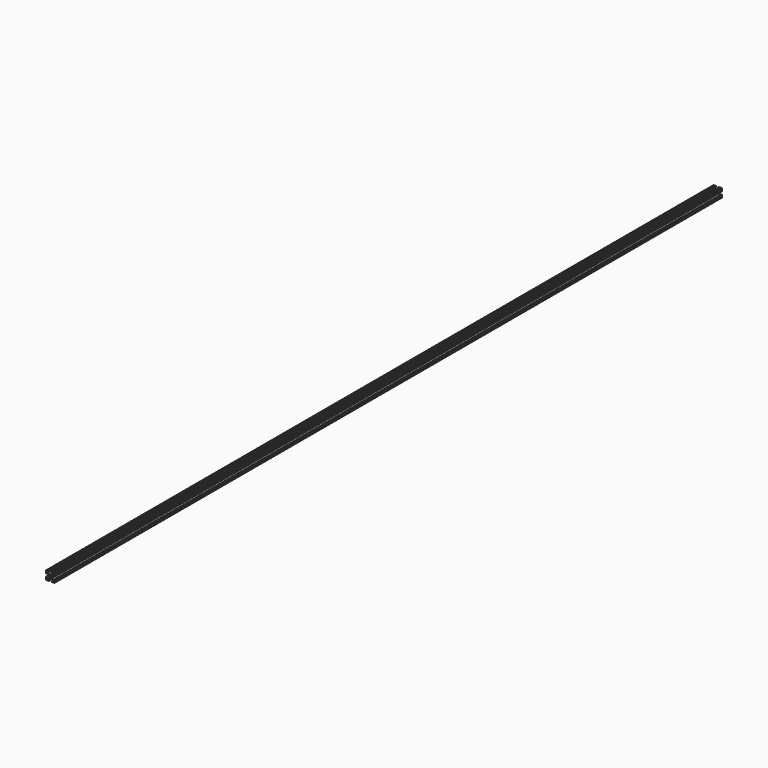
from build123d import *

# Parameters (mm, degrees)
F1_DEPTH    = 2438.4
F2_T1_DEPTH = 2438.4
F2_T3_DEPTH = 2446.3375
F2_T5_DEPTH = 2442.36875


# Not quite as in the source:
# - a fillet or chamfer that OpenCascade refuses, or shapes differently, is made with other operations: its cross-section is extruded or revolved along the edge and cut away or added


with BuildPart() as f1:
    # F0 (on Front) → F1 (new body)
    with BuildSketch(Plane.XZ):
        with BuildLine():
            ThreePointArc((-0.8361427067, 2.2296225996), (0, 2.38125), (0.8361427067, 2.2296225996))
            Line((0.8361427067, 2.2296225996), (3.1853789104, 4.5640625))
            Line((3.1853789104, 4.5640625), (-3.1853789104, 4.5640625))
            Line((-3.1853789104, 4.5640625), (-0.8361427067, 2.2296225996))
        make_face()
        with BuildLine():
            ThreePointArc((-2.2347427098, 0.8223603732), (-1.6889881746, 1.6785918231), (-0.8361427067, 2.2296225996))
            Line((-0.8361427067, 2.2296225996), (-3.1853789104, 4.5640625))
            Line((-3.1853789104, 4.5640625), (-4.5640625, 4.5640625))
            Line((-4.5640625, 4.5640625), (-4.5640625, 3.1376763557))
            Line((-4.5640625, 3.1376763557), (-2.2347427098, 0.8223603732))
        make_face()
        with BuildLine():
            ThreePointArc((-2.2347427098, -0.8223603732), (-2.38125, 0), (-2.2347427098, 0.8223603732))
            Line((-2.2347427098, 0.8223603732), (-4.5640625, 3.1376763557))
            Line((-4.5640625, 3.1376763557), (-4.5640625, -3.1376763557))
            Line((-4.5640625, -3.1376763557), (-2.2347427098, -0.8223603732))
        make_face()
        with BuildLine():
            Line((-3.1853789104, -4.5640625), (-0.8361427067, -2.2296225996))
            ThreePointArc((-0.8361427067, -2.2296225996), (-1.6889881746, -1.6785918231), (-2.2347427098, -0.8223603732))
            Line((-2.2347427098, -0.8223603732), (-4.5640625, -3.1376763557))
            Line((-4.5640625, -3.1376763557), (-4.5640625, -4.5640625))
            Line((-4.5640625, -4.5640625), (-3.1853789104, -4.5640625))
        make_face()
        with BuildLine():
            Line((3.1853789104, -4.5640625), (0.8361427067, -2.2296225996))
            ThreePointArc((0.8361427067, -2.2296225996), (0, -2.38125), (-0.8361427067, -2.2296225996))
            Line((-0.8361427067, -2.2296225996), (-3.1853789104, -4.5640625))
            Line((-3.1853789104, -4.5640625), (3.1853789104, -4.5640625))
        make_face()
        with BuildLine():
            Line((4.5640625, -3.1376763557), (2.2347427098, -0.8223603732))
            ThreePointArc((2.2347427098, -0.8223603732), (1.6889881746, -1.6785918231), (0.8361427067, -2.2296225996))
            Line((0.8361427067, -2.2296225996), (3.1853789104, -4.5640625))
            Line((3.1853789104, -4.5640625), (4.5640625, -4.5640625))
            Line((4.5640625, -4.5640625), (4.5640625, -3.1376763557))
        make_face()
        with BuildLine():
            ThreePointArc((2.2347427098, 0.8223603732), (2.3443370748, 0.4176544533), (2.38125, 0))
            ThreePointArc((2.38125, 0), (2.3443370748, -0.4176544533), (2.2347427098, -0.8223603732))
            Line((2.2347427098, -0.8223603732), (4.5640625, -3.1376763557))
            Line((4.5640625, -3.1376763557), (4.5640625, 3.1376763557))
            Line((4.5640625, 3.1376763557), (2.2347427098, 0.8223603732))
        make_face()
        with BuildLine():
            ThreePointArc((0.8361427067, 2.2296225996), (1.6889881746, 1.6785918231), (2.2347427098, 0.8223603732))
            Line((2.2347427098, 0.8223603732), (4.5640625, 3.1376763557))
            Line((4.5640625, 3.1376763557), (4.5640625, 4.5640625))
            Line((4.5640625, 4.5640625), (3.1853789104, 4.5640625))
            Line((3.1853789104, 4.5640625), (0.8361427067, 2.2296225996))
        make_face()
        Polygon((4.5640625, 4.5640625), (4.5640625, 3.1376763557), (10.715625, 9.2522558281), (12.7, 11.2247008192), (12.7, 12.7), (11.3728841543, 12.7), (9.3759316558, 10.715625), (3.1853789104, 4.5640625), align=None)
        with BuildLine():
            Line((12.7, 11.2247008192), (10.715625, 9.2522558281))
            Line((10.715625, 9.2522558281), (10.715625, 7.14375))
            Line((10.715625, 7.14375), (10.715625, 3.175))
            Line((10.715625, 3.175), (12.7, 3.175))
            Line((12.7, 3.175), (12.7, 5.55625))
            ThreePointArc((12.7, 5.55625), (12.303125, 5.953125), (12.7, 6.35))
            Line((12.7, 6.35), (12.7, 9.525))
            ThreePointArc((12.7, 9.525), (12.303125, 9.921875), (12.7, 10.31875))
            Line((12.7, 10.31875), (12.7, 11.2247008192))
        make_face()
        with BuildLine():
            Line((7.14375, 10.715625), (9.3759316558, 10.715625))
            Line((9.3759316558, 10.715625), (11.3728841543, 12.7))
            Line((11.3728841543, 12.7), (10.31875, 12.7))
            ThreePointArc((10.31875, 12.7), (9.921875, 12.303125), (9.525, 12.7))
            Line((9.525, 12.7), (6.35, 12.7))
            ThreePointArc((6.35, 12.7), (5.953125, 12.303125), (5.55625, 12.7))
            Line((5.55625, 12.7), (3.175, 12.7))
            Line((3.175, 12.7), (3.175, 10.715625))
            Line((3.175, 10.715625), (7.14375, 10.715625))
        make_face()
        with BuildLine():
            Line((-11.3728841543, 12.7), (-9.3759316558, 10.715625))
            Line((-9.3759316558, 10.715625), (-7.14375, 10.715625))
            Line((-7.14375, 10.715625), (-3.175, 10.715625))
            Line((-3.175, 10.715625), (-3.175, 12.7))
            Line((-3.175, 12.7), (-5.55625, 12.7))
            ThreePointArc((-5.55625, 12.7), (-5.953125, 12.303125), (-6.35, 12.7))
            Line((-6.35, 12.7), (-7.14375, 12.7))
            Line((-7.14375, 12.7), (-9.525, 12.7))
            ThreePointArc((-9.525, 12.7), (-9.921875, 12.303125), (-10.31875, 12.7))
            Line((-10.31875, 12.7), (-11.3728841543, 12.7))
        make_face()
        Polygon((-4.5640625, 4.5640625), (-3.1853789104, 4.5640625), (-9.3759316558, 10.715625), (-11.3728841543, 12.7), (-12.7, 11.2247008192), (-10.715625, 9.2522558281), (-4.5640625, 3.1376763557), align=None)
        Polygon((-12.7, 11.2247008192), (-11.3728841543, 12.7), (-12.7, 12.7), align=None)
        with BuildLine():
            Line((-10.715625, 7.14375), (-10.715625, 9.2522558281))
            Line((-10.715625, 9.2522558281), (-12.7, 11.2247008192))
            Line((-12.7, 11.2247008192), (-12.7, 10.31875))
            ThreePointArc((-12.7, 10.31875), (-12.303125, 9.921875), (-12.7, 9.525))
            Line((-12.7, 9.525), (-12.7, 6.35))
            ThreePointArc((-12.7, 6.35), (-12.303125, 5.953125), (-12.7, 5.55625))
            Line((-12.7, 5.55625), (-12.7, 3.175))
            Line((-12.7, 3.175), (-10.715625, 3.175))
            Line((-10.715625, 3.175), (-10.715625, 7.14375))
        make_face()
        with BuildLine():
            Line((-12.7, -11.2247008192), (-10.715625, -9.2522558281))
            Line((-10.715625, -9.2522558281), (-10.715625, -7.14375))
            Line((-10.715625, -7.14375), (-10.715625, -3.175))
            Line((-10.715625, -3.175), (-12.7, -3.175))
            Line((-12.7, -3.175), (-12.7, -5.55625))
            ThreePointArc((-12.7, -5.55625), (-12.303125, -5.953125), (-12.7, -6.35))
            Line((-12.7, -6.35), (-12.7, -9.525))
            ThreePointArc((-12.7, -9.525), (-12.303125, -9.921875), (-12.7, -10.31875))
            Line((-12.7, -10.31875), (-12.7, -11.2247008192))
        make_face()
        Polygon((-9.3759316558, -10.715625), (-3.1853789104, -4.5640625), (-4.5640625, -4.5640625), (-4.5640625, -3.1376763557), (-10.715625, -9.2522558281), (-12.7, -11.2247008192), (-12.7, -12.7), (-11.3728841543, -12.7), align=None)
        with BuildLine():
            Line((-7.14375, -10.715625), (-9.3759316558, -10.715625))
            Line((-9.3759316558, -10.715625), (-11.3728841543, -12.7))
            Line((-11.3728841543, -12.7), (-10.31875, -12.7))
            ThreePointArc((-10.31875, -12.7), (-9.921875, -12.303125), (-9.525, -12.7))
            Line((-9.525, -12.7), (-6.35, -12.7))
            ThreePointArc((-6.35, -12.7), (-5.953125, -12.303125), (-5.55625, -12.7))
            Line((-5.55625, -12.7), (-3.175, -12.7))
            Line((-3.175, -12.7), (-3.175, -10.715625))
            Line((-3.175, -10.715625), (-7.14375, -10.715625))
        make_face()
        with BuildLine():
            Line((11.3728841543, -12.7), (9.3759316558, -10.715625))
            Line((9.3759316558, -10.715625), (7.14375, -10.715625))
            Line((7.14375, -10.715625), (3.175, -10.715625))
            Line((3.175, -10.715625), (3.175, -12.7))
            Line((3.175, -12.7), (5.55625, -12.7))
            ThreePointArc((5.55625, -12.7), (5.953125, -12.303125), (6.35, -12.7))
            Line((6.35, -12.7), (9.525, -12.7))
            ThreePointArc((9.525, -12.7), (9.921875, -12.303125), (10.31875, -12.7))
            Line((10.31875, -12.7), (11.3728841543, -12.7))
        make_face()
        Polygon((10.715625, -9.2522558281), (4.5640625, -3.1376763557), (4.5640625, -4.5640625), (3.1853789104, -4.5640625), (9.3759316558, -10.715625), (11.3728841543, -12.7), (12.7, -12.7), (12.7, -11.2247008192), align=None)
        with BuildLine():
            Line((10.715625, -7.14375), (10.715625, -9.2522558281))
            Line((10.715625, -9.2522558281), (12.7, -11.2247008192))
            Line((12.7, -11.2247008192), (12.7, -10.31875))
            ThreePointArc((12.7, -10.31875), (12.303125, -9.921875), (12.7, -9.525))
            Line((12.7, -9.525), (12.7, -6.35))
            ThreePointArc((12.7, -6.35), (12.303125, -5.953125), (12.7, -5.55625))
            Line((12.7, -5.55625), (12.7, -3.175))
            Line((12.7, -3.175), (10.715625, -3.175))
            Line((10.715625, -3.175), (10.715625, -7.14375))
        make_face()
    extrude(amount=F1_DEPTH)

    # F2: fillet of radius 1.5875 on 31 edges, made by hand

    # F2_s2 → F2_t1 (join)
    with BuildSketch(Plane.XZ):
        with BuildLine():
            ThreePointArc((-6.6451596968, 8.0020523886), (-6.9937960043, 9.7333175229), (-5.5261794807, 10.715625))
            Line((-5.5261794807, 10.715625), (-9.3759316558, 10.715625))
            Line((-9.3759316558, 10.715625), (-6.6451596968, 8.0020523886))
        make_face()
        with BuildLine():
            ThreePointArc((-8.0089825615, 6.5618856508), (-9.7378452755, 6.9017155215), (-10.715625, 5.4359742634))
            Line((-10.715625, 5.4359742634), (-10.715625, 9.2522558281))
            Line((-10.715625, 9.2522558281), (-8.0089825615, 6.5618856508))
        make_face()
        with BuildLine():
            ThreePointArc((5.5261794807, 10.715625), (6.9937960043, 9.7333175229), (6.6451596968, 8.0020523886))
            Line((6.6451596968, 8.0020523886), (9.3759316558, 10.715625))
            Line((9.3759316558, 10.715625), (5.5261794807, 10.715625))
        make_face()
        with BuildLine():
            ThreePointArc((8.0089825615, 6.5618856508), (9.7378452755, 6.9017155215), (10.715625, 5.4359742634))
            Line((10.715625, 5.4359742634), (10.715625, 9.2522558281))
            Line((10.715625, 9.2522558281), (8.0089825615, 6.5618856508))
        make_face()
        with BuildLine():
            ThreePointArc((10.715625, -5.4359742634), (9.7378452755, -6.9017155215), (8.0089825615, -6.5618856508))
            Line((8.0089825615, -6.5618856508), (10.715625, -9.2522558281))
            Line((10.715625, -9.2522558281), (10.715625, -5.4359742634))
        make_face()
        with BuildLine():
            ThreePointArc((6.6451596968, -8.0020523886), (6.9937960043, -9.7333175229), (5.5261794807, -10.715625))
            Line((5.5261794807, -10.715625), (9.3759316558, -10.715625))
            Line((9.3759316558, -10.715625), (6.6451596968, -8.0020523886))
        make_face()
        with BuildLine():
            ThreePointArc((-5.5261794807, -10.715625), (-6.9937960043, -9.7333175229), (-6.6451596968, -8.0020523886))
            Line((-6.6451596968, -8.0020523886), (-9.3759316558, -10.715625))
            Line((-9.3759316558, -10.715625), (-5.5261794807, -10.715625))
        make_face()
        with BuildLine():
            ThreePointArc((-8.0089825615, -6.5618856508), (-9.7378452755, -6.9017155215), (-10.715625, -5.4359742634))
            Line((-10.715625, -5.4359742634), (-10.715625, -9.2522558281))
            Line((-10.715625, -9.2522558281), (-8.0089825615, -6.5618856508))
        make_face()
        with BuildLine():
            ThreePointArc((-2.530750733, 4.5640625), (-3.1359432558, 4.6839459764), (-3.649730949, 5.0254898886))
            Line((-3.649730949, 5.0254898886), (-3.1853789104, 4.5640625))
            Line((-3.1853789104, 4.5640625), (-2.530750733, 4.5640625))
        make_face()
    extrude(amount=F2_T1_DEPTH)

    # F2_s4 → F2_t3 (cut)
    with BuildSketch(Plane.XZ.offset(-3.96875)):
        with BuildLine():
            ThreePointArc((-12.7, -11.1125), (-12.2350320151, -12.2350320151), (-11.1125, -12.7))
            Line((-11.1125, -12.7), (-12.7, -12.7))
            Line((-12.7, -12.7), (-12.7, -11.1125))
        make_face()
        with BuildLine():
            ThreePointArc((11.1125, -12.7), (12.2350320151, -12.2350320151), (12.7, -11.1125))
            Line((12.7, -11.1125), (12.7, -12.7))
            Line((12.7, -12.7), (11.1125, -12.7))
        make_face()
        with BuildLine():
            ThreePointArc((12.7, 11.1125), (12.2350320151, 12.2350320151), (11.1125, 12.7))
            Line((11.1125, 12.7), (12.7, 12.7))
            Line((12.7, 12.7), (12.7, 11.1125))
        make_face()
        with BuildLine():
            ThreePointArc((-12.7, 4.7625), (-12.2350320151, 3.6399679849), (-11.1125, 3.175))
            Line((-11.1125, 3.175), (-12.7, 3.175))
            Line((-12.7, 3.175), (-12.7, 4.7625))
        make_face()
        with BuildLine():
            ThreePointArc((-11.1125, -3.175), (-12.2350320151, -3.6399679849), (-12.7, -4.7625))
            Line((-12.7, -4.7625), (-12.7, -3.175))
            Line((-12.7, -3.175), (-11.1125, -3.175))
        make_face()
        with BuildLine():
            ThreePointArc((-12.303125, 3.175), (-11.1805929849, 3.6399679849), (-10.715625, 4.7625))
            Line((-10.715625, 4.7625), (-10.715625, 3.175))
            Line((-10.715625, 3.175), (-12.303125, 3.175))
        make_face()
        with BuildLine():
            ThreePointArc((-10.715625, -4.7625), (-11.1805929849, -3.6399679849), (-12.303125, -3.175))
            Line((-12.303125, -3.175), (-10.715625, -3.175))
            Line((-10.715625, -3.175), (-10.715625, -4.7625))
        make_face()
        with BuildLine():
            ThreePointArc((-3.175, -12.303125), (-3.6399679849, -11.1805929849), (-4.7625, -10.715625))
            Line((-4.7625, -10.715625), (-3.175, -10.715625))
            Line((-3.175, -10.715625), (-3.175, -12.303125))
        make_face()
        with BuildLine():
            ThreePointArc((-4.7625, -12.7), (-3.6399679849, -12.2350320151), (-3.175, -11.1125))
            Line((-3.175, -11.1125), (-3.175, -12.7))
            Line((-3.175, -12.7), (-4.7625, -12.7))
        make_face()
        with BuildLine():
            ThreePointArc((3.175, -11.1125), (3.6399679849, -12.2350320151), (4.7625, -12.7))
            Line((4.7625, -12.7), (3.175, -12.7))
            Line((3.175, -12.7), (3.175, -11.1125))
        make_face()
        with BuildLine():
            ThreePointArc((4.7625, -10.715625), (3.6399679849, -11.1805929849), (3.175, -12.303125))
            Line((3.175, -12.303125), (3.175, -10.715625))
            Line((3.175, -10.715625), (4.7625, -10.715625))
        make_face()
        with BuildLine():
            ThreePointArc((12.7, -4.7625), (12.2350320151, -3.6399679849), (11.1125, -3.175))
            Line((11.1125, -3.175), (12.7, -3.175))
            Line((12.7, -3.175), (12.7, -4.7625))
        make_face()
        with BuildLine():
            ThreePointArc((11.1125, 3.175), (12.2350320151, 3.6399679849), (12.7, 4.7625))
            Line((12.7, 4.7625), (12.7, 3.175))
            Line((12.7, 3.175), (11.1125, 3.175))
        make_face()
        with BuildLine():
            ThreePointArc((12.303125, -3.175), (11.1805929849, -3.6399679849), (10.715625, -4.7625))
            Line((10.715625, -4.7625), (10.715625, -3.175))
            Line((10.715625, -3.175), (12.303125, -3.175))
        make_face()
        with BuildLine():
            ThreePointArc((10.715625, 4.7625), (11.1805929849, 3.6399679849), (12.303125, 3.175))
            Line((12.303125, 3.175), (10.715625, 3.175))
            Line((10.715625, 3.175), (10.715625, 4.7625))
        make_face()
        with BuildLine():
            ThreePointArc((-4.7625, 10.715625), (-3.6399679849, 11.1805929849), (-3.175, 12.303125))
            Line((-3.175, 12.303125), (-3.175, 10.715625))
            Line((-3.175, 10.715625), (-4.7625, 10.715625))
        make_face()
        with BuildLine():
            ThreePointArc((-3.175, 11.1125), (-3.6399679849, 12.2350320151), (-4.7625, 12.7))
            Line((-4.7625, 12.7), (-3.175, 12.7))
            Line((-3.175, 12.7), (-3.175, 11.1125))
        make_face()
        with BuildLine():
            ThreePointArc((4.7625, 12.7), (3.6399679849, 12.2350320151), (3.175, 11.1125))
            Line((3.175, 11.1125), (3.175, 12.7))
            Line((3.175, 12.7), (4.7625, 12.7))
        make_face()
        with BuildLine():
            ThreePointArc((3.175, 12.303125), (3.6399679849, 11.1805929849), (4.7625, 10.715625))
            Line((4.7625, 10.715625), (3.175, 10.715625))
            Line((3.175, 10.715625), (3.175, 12.303125))
        make_face()
        with BuildLine():
            ThreePointArc((-11.1125, 12.7), (-12.2350320151, 12.2350320151), (-12.7, 11.1125))
            Line((-12.7, 11.1125), (-12.7, 12.7))
            Line((-12.7, 12.7), (-11.1125, 12.7))
        make_face()
    extrude(amount=F2_T3_DEPTH, mode=Mode.SUBTRACT)

    # F2_s6 → F2_t5 (cut)
    with BuildSketch(Plane.XZ.offset(-1.984375)):
        with BuildLine():
            ThreePointArc((-8.73125, 12.7), (-9.2332615786, 12.6185347357), (-9.68375, 12.3825))
            ThreePointArc((-9.68375, 12.3825), (-9.5668992086, 12.5225121043), (-9.525, 12.7))
            Line((-9.525, 12.7), (-8.73125, 12.7))
        make_face()
        with BuildLine():
            ThreePointArc((-10.16, 12.3825), (-10.6104884214, 12.6185347357), (-11.1125, 12.7))
            Line((-11.1125, 12.7), (-10.31875, 12.7))
            ThreePointArc((-10.31875, 12.7), (-10.2768507914, 12.5225121043), (-10.16, 12.3825))
        make_face()
    extrude(amount=F2_T5_DEPTH, mode=Mode.SUBTRACT)


solid = f1.part
